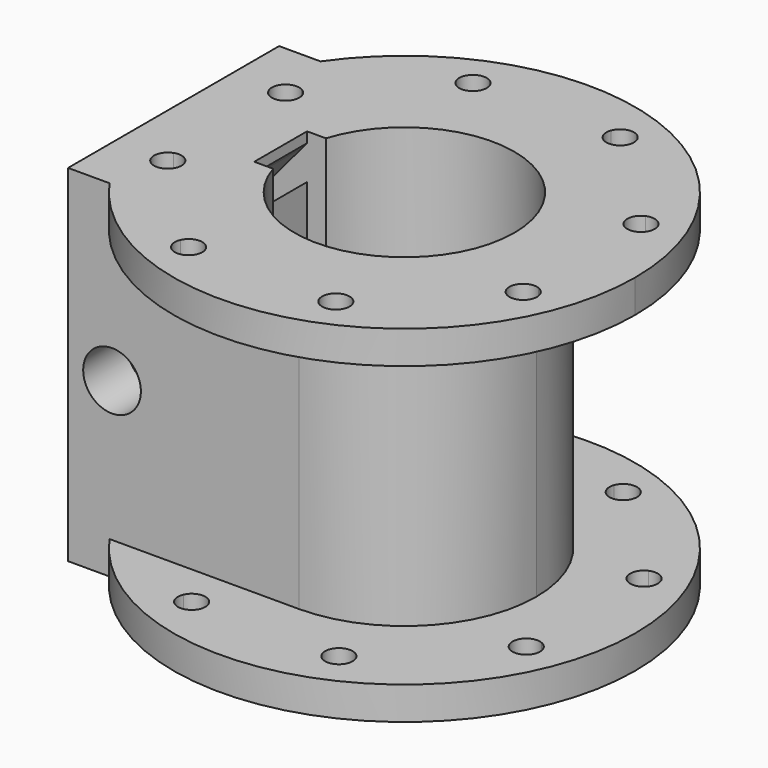
from build123d import *

# Parameters (mm, degrees)
F0_R           = 42
F1_DEPTH       = 6
F3_DEPTH       = 6
F4_DEPTH       = 57
F6_DEPTH       = 6
F8_D           = 40
F8_DEPTH       = 63
F8_CBORE_D     = 48
F8_CBORE_DEPTH = 3
F8_TIP         = 12.0172123806
F10_DEPTH      = 8
F11_DEPTH      = 10
F13_DEPTH      = 63.001
F16_DEPTH      = 15
F18_DEPTH      = 9.91
F20_DEPTH      = 6
F20_DEPTH_BACK = 6
F21_DEPTH      = 6
F22_DEPTH      = 25


# Not quite as in the source:
# - a feature names something its author has since deleted; it is built from what else it names


with BuildPart() as f1:
    # F0 (on Top) → F1 (new body)
    with BuildSketch(Plane.XY):
        Circle(F0_R)
    extrude(amount=F1_DEPTH)

    # F2 (on face) → F3 (join)
    with BuildSketch(Plane.XY.offset(6)):
        with BuildLine():
            ThreePointArc((-42, 0), (-40.072620247, 12.5771660773), (-34.4673758792, 24))
            Line((-34.4673758792, 24), (-42, 24))
            Line((-42, 24), (-42, 0))
        make_face()
        with BuildLine():
            Line((-42, -24), (-34.4673758792, -24))
            ThreePointArc((-34.4673758792, -24), (-40.072620247, -12.5771660773), (-42, 0))
            Line((-42, 0), (-42, -24))
        make_face()
    extrude(amount=-F3_DEPTH)

    # F2 (on face) → F4 (join)
    with BuildSketch(Plane.XY.offset(6)):
        with BuildLine():
            ThreePointArc((0, -24), (16.9705627485, -16.9705627485), (24, 0))
            ThreePointArc((24, 0), (16.9705627485, 16.9705627485), (0, 24))
            ThreePointArc((0, 24), (-24, 0), (0, -24))
        make_face()
        with BuildLine():
            ThreePointArc((0, -24), (-24, 0), (0, 24))
            Line((0, 24), (-34.4673758792, 24))
            ThreePointArc((-34.4673758792, 24), (-40.072620247, 12.5771660773), (-42, 0))
            ThreePointArc((-42, 0), (-40.072620247, -12.5771660773), (-34.4673758792, -24))
            Line((-34.4673758792, -24), (0, -24))
        make_face()
        with BuildLine():
            Line((-42, -24), (-34.4673758792, -24))
            ThreePointArc((-34.4673758792, -24), (-40.072620247, -12.5771660773), (-42, 0))
            Line((-42, 0), (-42, -24))
        make_face()
        with BuildLine():
            ThreePointArc((-42, 0), (-40.072620247, 12.5771660773), (-34.4673758792, 24))
            Line((-34.4673758792, 24), (-42, 24))
            Line((-42, 24), (-42, 0))
        make_face()
    extrude(amount=F4_DEPTH)

    # F5 (on face) → F6 (join)
    with BuildSketch(Plane.XY.offset(63)):
        with BuildLine():
            ThreePointArc((-34.4673758792, -24), (12.5771660773, -40.072620247), (42, 0))
            ThreePointArc((42, 0), (12.5771660773, 40.072620247), (-34.4673758792, 24))
            Line((-34.4673758792, 24), (0, 24))
            ThreePointArc((0, 24), (24, 0), (0, -24))
            Line((0, -24), (-34.4673758792, -24))
        make_face()
    extrude(amount=-F6_DEPTH)

    # F8
    with Locations(Plane(origin=(0, 0, 0), x_dir=(1, 0, 0), z_dir=(0, 0, -1))):
        with Locations((0, 0)):
            CounterBoreHole(F8_D / 2, F8_CBORE_D / 2, F8_CBORE_DEPTH, depth=F8_DEPTH)
            with Locations((0, 0, -(F8_DEPTH + F8_TIP / 2))):  # 118° drill point
                Cone(0, F8_D / 2, F8_TIP, mode=Mode.SUBTRACT)

    # F9 (on face) → F10 (cut)
    with BuildSketch(Plane(origin=(-42, 0, 0), x_dir=(0, -1, 0), z_dir=(-1, 0, 0))):
        with BuildLine():
            Line((12, 40.5), (-12, 40.5))
            ThreePointArc((-12, 40.5), (-14, 38.5), (-12, 36.5))
            Line((-12, 36.5), (12, 36.5))
            ThreePointArc((12, 36.5), (14, 38.5), (12, 40.5))
        make_face()
        with BuildLine():
            Line((12, 34.5), (-12, 34.5))
            ThreePointArc((-12, 34.5), (-15, 31.5), (-12, 28.5))
            Line((-12, 28.5), (12, 28.5))
            ThreePointArc((12, 28.5), (15, 31.5), (12, 34.5))
        make_face()
        with BuildLine():
            Line((12, 26.4393606186), (-12, 26.4393606186))
            ThreePointArc((-12, 26.4393606186), (-14, 24.4393606186), (-12, 22.4393606186))
            Line((-12, 22.4393606186), (12, 22.4393606186))
            ThreePointArc((12, 22.4393606186), (14, 24.4393606186), (12, 26.4393606186))
        make_face()
    extrude(amount=-F10_DEPTH, mode=Mode.SUBTRACT)

    # F9 (on face) → F11 (cut)
    with BuildSketch(Plane(origin=(-42, 0, 0), x_dir=(0, -1, 0), z_dir=(-1, 0, 0))):
        with BuildLine():
            ThreePointArc((-19, 6.65), (-20.166726189, 3.833273811), (-17.35, 5))
            Line((-17.35, 5), (-19, 5))
            Line((-19, 5), (-19, 6.65))
        make_face()
        with BuildLine():
            Line((-19, 5), (-17.35, 5))
            ThreePointArc((-17.35, 5), (-17.833273811, 6.166726189), (-19, 6.65))
            Line((-19, 6.65), (-19, 5))
        make_face()
        with BuildLine():
            Line((19, 6.65), (19, 5))
            Line((19, 5), (17.35, 5))
            ThreePointArc((17.35, 5), (19, 3.35), (20.65, 5))
            ThreePointArc((20.65, 5), (20.166726189, 6.166726189), (19, 6.65))
        make_face()
        with BuildLine():
            Line((17.35, 5), (19, 5))
            Line((19, 5), (19, 6.65))
            ThreePointArc((19, 6.65), (17.833273811, 6.166726189), (17.35, 5))
        make_face()
        with BuildLine():
            ThreePointArc((17.35, 58), (17.833273811, 56.833273811), (19, 56.35))
            Line((19, 56.35), (19, 58))
            Line((19, 58), (17.35, 58))
        make_face()
        with BuildLine():
            Line((19, 58), (19, 56.35))
            ThreePointArc((19, 56.35), (20.166726189, 56.833273811), (20.65, 58))
            ThreePointArc((20.65, 58), (19, 59.65), (17.35, 58))
            Line((17.35, 58), (19, 58))
        make_face()
        with BuildLine():
            ThreePointArc((-19, 56.35), (-17.833273811, 56.833273811), (-17.35, 58))
            Line((-17.35, 58), (-19, 58))
            Line((-19, 58), (-19, 56.35))
        make_face()
        with BuildLine():
            Line((-19, 58), (-17.35, 58))
            ThreePointArc((-17.35, 58), (-20.166726189, 59.166726189), (-19, 56.35))
            Line((-19, 56.35), (-19, 58))
        make_face()
    extrude(amount=-F11_DEPTH, mode=Mode.SUBTRACT)

    # F12 (on face) → F13 (cut, through all)
    with BuildSketch(Plane.XY.offset(63)):
        with BuildLine():
            Line((-19.0787840283, 6), (-20, 6))
            Line((-20, 6), (-22.5187840283, 6))
            Line((-22.5187840283, 6), (-22.5187840283, -6))
            Line((-22.5187840283, -6), (-20, -6))
            Line((-20, -6), (-19.0787840283, -6))
            ThreePointArc((-19.0787840283, -6), (-20, 0), (-19.0787840283, 6))
        make_face()
    extrude(amount=-F13_DEPTH, mode=Mode.SUBTRACT)

    # F15 (on face) → F16 (cut)
    with BuildSketch(Plane(origin=(0, 0, 0), x_dir=(1, 0, 0), z_dir=(0, 0, -1))):
        with BuildLine():
            ThreePointArc((31.4161860333, 15.1226736182), (30.1450746865, 11.8919078618), (33.3283825142, 10.5062229401))
            ThreePointArc((33.3283825142, 10.5062229401), (32.4547735177, 12.8486164427), (31.4161860333, 15.1226736182))
        make_face()
        with BuildLine():
            ThreePointArc((31.4161860333, 15.1226736182), (32.4547735177, 12.8486164427), (33.3283825142, 10.5062229401))
            ThreePointArc((33.3283825142, 10.5062229401), (34.5083097959, 11.4227872965), (34.9547735177, 12.8486164427))
            ThreePointArc((34.9547735177, 12.8486164427), (33.8063524627, 14.9517651193), (31.4161860333, 15.1226736182))
        make_face()
        with BuildLine():
            ThreePointArc((34.9547735177, -13.9392238228), (34.5083097959, -12.5133946765), (33.3283825142, -11.5968303202))
            ThreePointArc((33.3283825142, -11.5968303202), (32.4547735177, -13.9392238228), (31.4161860333, -16.2132809983))
            ThreePointArc((31.4161860333, -16.2132809983), (33.8063524627, -16.0423724993), (34.9547735177, -13.9392238228))
        make_face()
        with BuildLine():
            ThreePointArc((31.4161860333, -16.2132809983), (32.4547735177, -13.9392238228), (33.3283825142, -11.5968303202))
            ThreePointArc((33.3283825142, -11.5968303202), (30.1450746865, -12.9825152419), (31.4161860333, -16.2132809983))
        make_face()
        with BuildLine():
            ThreePointArc((11.17051651, 32.6640889443), (12.5562014317, 29.4807811166), (15.7869671881, 30.7518924634))
            ThreePointArc((15.7869671881, 30.7518924634), (13.5129100126, 31.7904799479), (11.17051651, 32.6640889443))
        make_face()
        with BuildLine():
            ThreePointArc((11.17051651, 32.6640889443), (13.5129100126, 31.7904799479), (15.7869671881, 30.7518924634))
            ThreePointArc((15.7869671881, 30.7518924634), (15.9557713409, 31.2590398941), (16.0129100126, 31.7904799479))
            ThreePointArc((16.0129100126, 31.7904799479), (13.9567659822, 34.2507628337), (11.17051651, 32.6640889443))
        make_face()
        with BuildLine():
            ThreePointArc((16.0129100126, -32.8810873279), (15.9557713409, -32.3496472742), (15.7869671881, -31.8424998435))
            ThreePointArc((15.7869671881, -31.8424998435), (13.5129100126, -32.8810873279), (11.17051651, -33.7546963244))
            ThreePointArc((11.17051651, -33.7546963244), (13.9567659822, -35.3413702138), (16.0129100126, -32.8810873279))
        make_face()
        with BuildLine():
            ThreePointArc((11.17051651, -33.7546963244), (13.5129100126, -32.8810873279), (15.7869671881, -31.8424998435))
            ThreePointArc((15.7869671881, -31.8424998435), (12.5562014317, -30.5713884966), (11.17051651, -33.7546963244))
        make_face()
        with BuildLine():
            ThreePointArc((-10.7749302529, 31.7904799479), (-10.8146473671, 32.2343359174), (-10.9325367503, 32.6640889443))
            ThreePointArc((-10.9325367503, 32.6640889443), (-13.2749302529, 31.7904799479), (-15.5489874284, 30.7518924634))
            ThreePointArc((-15.5489874284, 30.7518924634), (-12.7434901992, 29.3476186196), (-10.7749302529, 31.7904799479))
        make_face()
        with BuildLine():
            ThreePointArc((-15.5489874284, 30.7518924634), (-13.2749302529, 31.7904799479), (-10.9325367503, 32.6640889443))
            ThreePointArc((-10.9325367503, 32.6640889443), (-14.2316388338, 34.1001787791), (-15.5489874284, 30.7518924634))
        make_face()
        with BuildLine():
            ThreePointArc((-15.5489874284, -31.8424998435), (-14.2316388338, -35.1907861592), (-10.9325367503, -33.7546963244))
            ThreePointArc((-10.9325367503, -33.7546963244), (-13.2749302529, -32.8810873279), (-15.5489874284, -31.8424998435))
        make_face()
        with BuildLine():
            ThreePointArc((-15.5489874284, -31.8424998435), (-13.2749302529, -32.8810873279), (-10.9325367503, -33.7546963244))
            ThreePointArc((-10.9325367503, -33.7546963244), (-10.8146473671, -33.3249432975), (-10.7749302529, -32.8810873279))
            ThreePointArc((-10.7749302529, -32.8810873279), (-12.7434901992, -30.4382259996), (-15.5489874284, -31.8424998435))
        make_face()
        with BuildLine():
            ThreePointArc((-29.716793758, 12.8486164427), (-30.1136450815, 14.2001953877), (-31.1782062736, 15.1226736182))
            ThreePointArc((-31.1782062736, 15.1226736182), (-31.7178105764, 13.9949210919), (-32.216793758, 12.8486164427))
            Line((-32.216793758, 12.8486164427), (-29.9070949268, 11.8919078618))
            ThreePointArc((-29.9070949268, 11.8919078618), (-29.764830557, 12.3608906377), (-29.716793758, 12.8486164427))
        make_face()
        with BuildLine():
            ThreePointArc((-32.216793758, 12.8486164427), (-31.7178105764, 13.9949210919), (-31.1782062736, 15.1226736182))
            ThreePointArc((-31.1782062736, 15.1226736182), (-33.13209854, 15.1750336788), (-34.5264925893, 13.8053250237))
            Line((-34.5264925893, 13.8053250237), (-32.216793758, 12.8486164427))
        make_face()
        with BuildLine():
            ThreePointArc((-33.0904027545, -11.5968303202), (-34.5264925893, -14.8959324037), (-31.1782062736, -16.2132809983))
            ThreePointArc((-31.1782062736, -16.2132809983), (-32.216793758, -13.9392238228), (-33.0904027545, -11.5968303202))
        make_face()
        with BuildLine():
            ThreePointArc((-33.0904027545, -11.5968303202), (-32.216793758, -13.9392238228), (-31.1782062736, -16.2132809983))
            ThreePointArc((-31.1782062736, -16.2132809983), (-30.1136450815, -15.2908027678), (-29.716793758, -13.9392238228))
            ThreePointArc((-29.716793758, -13.9392238228), (-30.7909646118, -11.8856875447), (-33.0904027545, -11.5968303202))
        make_face()
        with BuildLine():
            Line((-29.9070949268, 11.8919078618), (-32.216793758, 12.8486164427))
            ThreePointArc((-32.216793758, 12.8486164427), (-32.6745191573, 11.6852222606), (-33.0904027545, 10.5062229401))
            ThreePointArc((-33.0904027545, 10.5062229401), (-31.2189865728, 10.5563728211), (-29.9070949268, 11.8919078618))
        make_face()
        with BuildLine():
            ThreePointArc((-33.0904027545, 10.5062229401), (-32.6745191573, 11.6852222606), (-32.216793758, 12.8486164427))
            Line((-32.216793758, 12.8486164427), (-34.5264925893, 13.8053250237))
            ThreePointArc((-34.5264925893, 13.8053250237), (-34.5090373797, 11.8508092575), (-33.0904027545, 10.5062229401))
        make_face()
    extrude(amount=-F16_DEPTH, mode=Mode.SUBTRACT)

    # F17 (on face) → F18 (cut)
    with BuildSketch(Plane.XZ.offset(24)):
        with BuildLine():
            ThreePointArc((-28.75, 31.5), (-34, 36.75), (-39.25, 31.5))
            ThreePointArc((-39.25, 31.5), (-34, 26.25), (-28.75, 31.5))
        make_face()
    extrude(amount=-F18_DEPTH, mode=Mode.SUBTRACT)

    # F19 (on Front) → F20 (cut, two sides)
    with BuildSketch(Plane.XZ) as f20_sk:
        Polygon((-39.1897655987, 21.7698397348), (-24.0202943734, 3.6915679043), (-23.7301471867, 3.3457839522), (-21.8293532023, 3.3457839522), (-21.8293532023, 7.3034011999), (-23.44, 9.2228953074), (-31.7884148034, 19.1721486418), (-36.259012913, 24.5), (-41.4806420703, 24.5), align=None)
        Polygon((-41.4806420703, 38.5), (-36.259012913, 38.5), (-23.44, 53.7771046926), (-21.8293532023, 55.6965988001), (-21.8293532023, 61.9194941076), (-23.44, 60), (-39.1897655987, 41.2301602652), align=None)
    extrude(amount=-F20_DEPTH, mode=Mode.SUBTRACT)
    extrude(f20_sk.sketch, amount=F20_DEPTH_BACK, mode=Mode.SUBTRACT)

    # F19 (on Front) → F21 (cut, through all)
    with BuildSketch(Plane.XZ):
        Polygon((-39.1897655987, 21.7698397348), (-24.0202943734, 3.6915679043), (-23.7301471867, 3.3457839522), (-21.8293532023, 3.3457839522), (-21.8293532023, 7.3034011999), (-23.44, 9.2228953074), (-31.7884148034, 19.1721486418), (-36.259012913, 24.5), (-41.4806420703, 24.5), align=None)
        Polygon((-41.4806420703, 38.5), (-36.259012913, 38.5), (-23.44, 53.7771046926), (-21.8293532023, 55.6965988001), (-21.8293532023, 61.9194941076), (-23.44, 60), (-39.1897655987, 41.2301602652), align=None)
    extrude(amount=F21_DEPTH, mode=Mode.SUBTRACT)

    # F14 (on face) → F22 (cut)
    with BuildSketch(Plane.XY.offset(63)):
        with BuildLine():
            ThreePointArc((11.0515266301, -33.2093926344), (13.3939201328, -32.3357836379), (15.6679773082, -31.2971961535))
            ThreePointArc((15.6679773082, -31.2971961535), (12.4372115519, -30.0260848066), (11.0515266301, -33.2093926344))
        make_face()
        with BuildLine():
            ThreePointArc((15.8939201328, -32.3357836379), (15.8367814611, -31.8043435842), (15.6679773082, -31.2971961535))
            ThreePointArc((15.6679773082, -31.2971961535), (13.3939201328, -32.3357836379), (11.0515266301, -33.2093926344))
            ThreePointArc((11.0515266301, -33.2093926344), (13.8377761023, -34.7960665237), (15.8939201328, -32.3357836379))
        make_face()
        with BuildLine():
            ThreePointArc((34.8357836379, -13.3939201328), (34.389319916, -11.9680909865), (33.2093926344, -11.0515266301))
            ThreePointArc((33.2093926344, -11.0515266301), (32.3357836379, -13.3939201328), (31.2971961535, -15.6679773082))
            ThreePointArc((31.2971961535, -15.6679773082), (33.6873625829, -15.4970688093), (34.8357836379, -13.3939201328))
        make_face()
        with BuildLine():
            ThreePointArc((31.2971961535, -15.6679773082), (32.3357836379, -13.3939201328), (33.2093926344, -11.0515266301))
            ThreePointArc((33.2093926344, -11.0515266301), (30.0260848066, -12.4372115519), (31.2971961535, -15.6679773082))
        make_face()
        with BuildLine():
            ThreePointArc((31.2971961535, 15.6679773082), (30.0260848066, 12.4372115519), (33.2093926344, 11.0515266301))
            ThreePointArc((33.2093926344, 11.0515266301), (32.3357836379, 13.3939201328), (31.2971961535, 15.6679773082))
        make_face()
        with BuildLine():
            ThreePointArc((31.2971961535, 15.6679773082), (32.3357836379, 13.3939201328), (33.2093926344, 11.0515266301))
            ThreePointArc((33.2093926344, 11.0515266301), (34.389319916, 11.9680909865), (34.8357836379, 13.3939201328))
            ThreePointArc((34.8357836379, 13.3939201328), (33.6873625829, 15.4970688093), (31.2971961535, 15.6679773082))
        make_face()
        with BuildLine():
            ThreePointArc((11.0515266301, 33.2093926344), (12.4372115519, 30.0260848066), (15.6679773082, 31.2971961535))
            ThreePointArc((15.6679773082, 31.2971961535), (13.3939201328, 32.3357836379), (11.0515266301, 33.2093926344))
        make_face()
        with BuildLine():
            ThreePointArc((11.0515266301, 33.2093926344), (13.3939201328, 32.3357836379), (15.6679773082, 31.2971961535))
            ThreePointArc((15.6679773082, 31.2971961535), (15.8367814611, 31.8043435842), (15.8939201328, 32.3357836379))
            ThreePointArc((15.8939201328, 32.3357836379), (13.8377761023, 34.7960665237), (11.0515266301, 33.2093926344))
        make_face()
        with BuildLine():
            ThreePointArc((-15.6679773082, 31.2971961535), (-13.3939201328, 32.3357836379), (-11.0515266301, 33.2093926344))
            ThreePointArc((-11.0515266301, 33.2093926344), (-14.3506287137, 34.6454824692), (-15.6679773082, 31.2971961535))
        make_face()
        with BuildLine():
            ThreePointArc((-10.8939201328, 32.3357836379), (-10.9336372469, 32.7796396074), (-11.0515266301, 33.2093926344))
            ThreePointArc((-11.0515266301, 33.2093926344), (-13.3939201328, 32.3357836379), (-15.6679773082, 31.2971961535))
            ThreePointArc((-15.6679773082, 31.2971961535), (-12.8624800791, 29.8929223096), (-10.8939201328, 32.3357836379))
        make_face()
        with BuildLine():
            ThreePointArc((-15.6679773082, -31.2971961535), (-14.3506287137, -34.6454824692), (-11.0515266301, -33.2093926344))
            ThreePointArc((-11.0515266301, -33.2093926344), (-13.3939201328, -32.3357836379), (-15.6679773082, -31.2971961535))
        make_face()
        with BuildLine():
            ThreePointArc((-15.6679773082, -31.2971961535), (-13.3939201328, -32.3357836379), (-11.0515266301, -33.2093926344))
            ThreePointArc((-11.0515266301, -33.2093926344), (-10.9336372469, -32.7796396074), (-10.8939201328, -32.3357836379))
            ThreePointArc((-10.8939201328, -32.3357836379), (-12.8624800791, -29.8929223096), (-15.6679773082, -31.2971961535))
        make_face()
        with BuildLine():
            ThreePointArc((-33.2093926344, -11.0515266301), (-32.3357836379, -13.3939201328), (-31.2971961535, -15.6679773082))
            ThreePointArc((-31.2971961535, -15.6679773082), (-30.2326349614, -14.7454990777), (-29.8357836379, -13.3939201328))
            ThreePointArc((-29.8357836379, -13.3939201328), (-30.9099544916, -11.3403838546), (-33.2093926344, -11.0515266301))
        make_face()
        with BuildLine():
            ThreePointArc((-33.2093926344, -11.0515266301), (-34.6454824692, -14.3506287137), (-31.2971961535, -15.6679773082))
            ThreePointArc((-31.2971961535, -15.6679773082), (-32.3357836379, -13.3939201328), (-33.2093926344, -11.0515266301))
        make_face()
        with BuildLine():
            ThreePointArc((-29.8357836379, 13.3939201328), (-30.2326349614, 14.7454990777), (-31.2971961535, 15.6679773082))
            ThreePointArc((-31.2971961535, 15.6679773082), (-32.3357836379, 13.3939201328), (-33.2093926344, 11.0515266301))
            ThreePointArc((-33.2093926344, 11.0515266301), (-30.9099544916, 11.3403838546), (-29.8357836379, 13.3939201328))
        make_face()
        with BuildLine():
            ThreePointArc((-33.2093926344, 11.0515266301), (-32.3357836379, 13.3939201328), (-31.2971961535, 15.6679773082))
            ThreePointArc((-31.2971961535, 15.6679773082), (-34.6454824692, 14.3506287137), (-33.2093926344, 11.0515266301))
        make_face()
    extrude(amount=-F22_DEPTH, mode=Mode.SUBTRACT)


solid = f1.part
